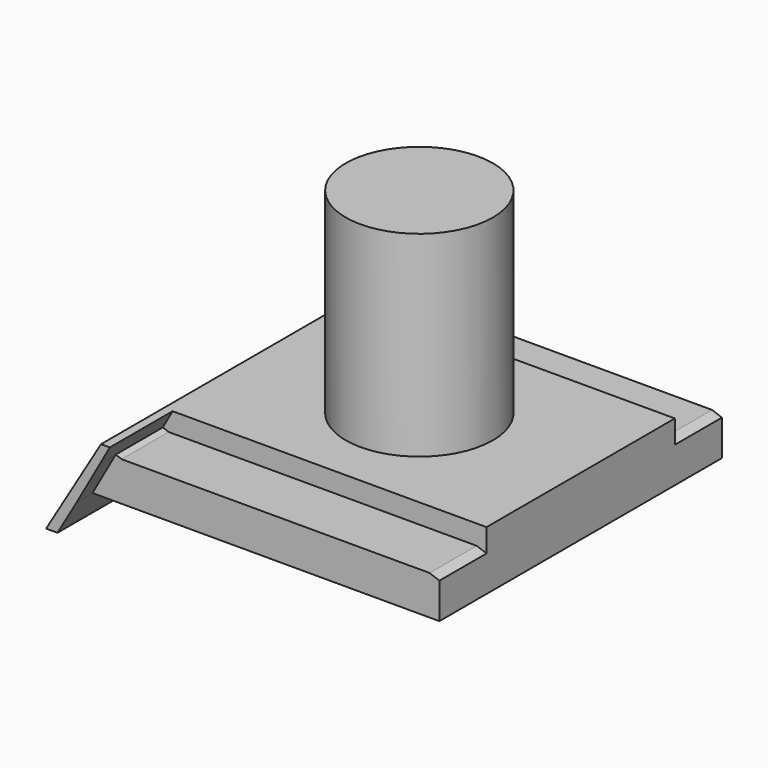
from build123d import *

# Parameters (mm, degrees)
F1_DEPTH  = 20
F3_DEPTH  = 4
F5_DEPTH  = 1
F7_DEPTH  = 20.001
F10_W     = 15
F10_H     = 9.1
F11_DEPTH = 1
F8_R      = 3.75
F12_DEPTH = 10


# Not quite as in the source:
# - a pattern or mirror of a feature is missing from the dataset's text; its kind, count and spacing are read off the source's solid


with BuildPart() as f1:
    # F0 (on Front) → F1 (new body)
    with BuildSketch(Plane.XZ):
        Polygon((-16.45, 3), (-19.25, -1.7), (-18.09, -1.7), (-17.0772340426, 0), (0, 0), (0, 3), align=None)
    extrude(amount=F1_DEPTH)

    # F2 (on face) → F3 (cut)
    with BuildSketch(Plane.XZ.offset(20)):
        Polygon((-16.2, 2), (-0.5, 2), (0, 1.8180148829), (0, 3), (-16, 3), (-16.5, 2.1091910703), align=None)
    f3 = extrude(amount=-F3_DEPTH, mode=Mode.SUBTRACT)

    # F3_copies: F3 across plane
    add(f3.mirror(Plane.ZX.offset(-10)), mode=Mode.SUBTRACT)

    # F4 (on face) → F5 (cut)
    with BuildSketch(Plane.XZ.offset(20)):
        Polygon((0, 0), (0, 1.8180148829), (-0.5, 2), (-16.2, 2), (-16.5, 2.1091910703), (-17.683862779, 0), align=None)
    f5 = extrude(amount=-F5_DEPTH, mode=Mode.SUBTRACT)

    # F5_copies: F5 across plane
    add(f5.mirror(Plane.ZX.offset(-10)), mode=Mode.SUBTRACT)

    # F6 (on face) → F7 (cut, through all)
    with BuildSketch(Plane.XZ.offset(20)):
        Polygon((-18.67, -1.7), (-18.09, -1.7), (-17.0772340426, 0), (-17.683862779, 0), align=None)
    extrude(amount=-F7_DEPTH, mode=Mode.SUBTRACT)

    # F10 (on face) → F11 (cut)
    with BuildSketch(Plane(origin=(0, 0, 0), x_dir=(1, 0, 0), z_dir=(0, 0, -1))):
        with Locations((-9, 10)):
            Rectangle(F10_W, F10_H)
    extrude(amount=-F11_DEPTH, mode=Mode.SUBTRACT)

    # F8 (on face) → F12 (join)
    with BuildSketch(Plane.XY.offset(3)):
        with Locations((-8.225, -10)):
            Circle(F8_R)
    extrude(amount=F12_DEPTH)


solid = f1.part
